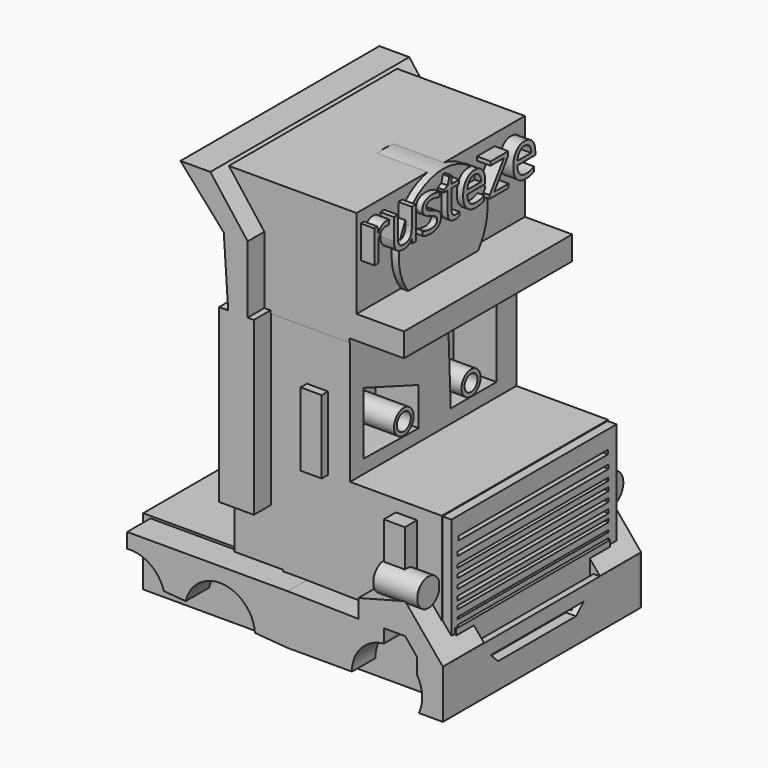
from build123d import *

# Parameters (mm, degrees)
F1_DEPTH       = 38.862
F1_DEPTH_BACK  = 39.878
F2_W           = 20.1118066907
F2_H           = 32.6452478766
F2_W_2         = 7.5783613138
F3_DEPTH       = 31.242
F3_DEPTH_BACK  = 34.798
F4_W           = 6.7039392889
F4_H           = 21.5691800695
F5_DEPTH       = 36.068
F5_DEPTH_BACK  = 37.084
F6_W           = 6.7039350979
F6_H           = 23.3180318028
F7_DEPTH       = 33.782
F7_DEPTH_BACK  = 36.83
F8_W           = 15.4481963255
F8_H           = 23.6095087603
F8_H_2         = 47.5104935467
F9_DEPTH       = 31.242
F9_DEPTH_BACK  = 35.052
F11_DEPTH      = 38.1
F11_DEPTH_BACK = 40.894
F13_DEPTH      = 31.496
F13_DEPTH_BACK = 35.306
F14_W          = 46.0130926222
F14_H          = 31.2351649627
F15_DEPTH      = 104.902
F15_DEPTH_BACK = 66.294
F16_R          = 11.155404916
F17_DEPTH      = 52.578
F17_DEPTH_BACK = 51.308
F18_R          = 3.81
F19_DEPTH      = 49.022
F19_DEPTH_BACK = 51.562
F20_DEPTH      = 25.4
F21_TEXT_SIZE  = 19.3375005654
F22_DEPTH      = 4.318
F23_R          = 17.6319533446
F24_DEPTH      = 18.288
F26_DEPTH      = 29.718
F27_R          = 3.8767676241
F27_R_2        = 2.7666686099
F27_R_3        = 3.7900369815
F27_R_4        = 2.5845106844
F28_DEPTH      = 13.716
F30_START      = 27.94
F29_R          = 4.4370042328
F29_R_2        = 4.9895919821
F30_DEPTH      = 13.97
F32_START      = 42.418
F31_W          = 65.579129383
F31_H          = 43.979652226
F32_DEPTH      = 3.302
F33_W          = 59.333499521
F33_H          = 1.3011721894
F33_W_2        = 60.1142030209
F33_H_2        = 1.3011731207
F33_H_3        = 0.9682839736
F33_H_4        = 1.1880891398
F33_H_5        = 1.1880899547
F33_H_6        = 1.2545959326
F33_H_7        = 1.0560783558
F33_H_8        = 0.660049729
F33_H_9        = 0.765087083
F34_DEPTH      = 11.176
F34_DEPTH_BACK = 4.064
F35_DEPTH      = 14.478
F37_START      = 47.244
F36_W          = 77.5241665542
F36_H          = 24.3252208456
F37_DEPTH      = 2.032
F38_W          = 9.0682730079
F38_H          = 14.4420657307
F39_DEPTH      = 40.894
F39_DEPTH_BACK = 39.37
F40_W          = 103.7813574076
F40_H          = 8.3965491503
F41_DEPTH      = 22.606
F41_DEPTH_BACK = 24.13
F42_W          = 36.1429508775
F42_H          = 4.5344494283
F43_DEPTH      = 0.254
F43_DEPTH_BACK = 66.04
F44_R          = 1.27
F45_DEPTH      = 41.91
F47_START      = 44.704
F47_DEPTH      = 21.336
F48_W          = 46.3489554822
F48_H          = 29.5391734689
F49_DEPTH      = 22.86
F51_START      = -8.636
F50_W          = 99.3931107223
F50_H          = 61.2098351121
F51_DEPTH      = 21.336


# Not quite as in the source:
# - Text() gives the source's letters only with a copy of the font that has no kerning and outlines rounded to 1/6400 em; it was checked with that copy


with BuildPart() as f1:
    # F0 (on Front) → F1 (new body, two sides)
    with BuildSketch(Plane.XZ) as f1_sk:
        Polygon((22.4436074495, -25.212623179), (30.3134415299, -25.212623179), (30.6049156934, -9.7644263878), (37.3088568449, -9.7644263878), (41.098035872, -14.4280325621), (41.098035872, -34.5398373902), (49.2593459785, -39.2034426332), (49.2593459785, -14.4280325621), (37.3088568449, 0), (22.4436074495, -3.9349179715), (22.4436074495, -9.7644263878), align=None)
        Polygon((0, -25.212623179), (22.4436074495, -25.212623179), (22.4436074495, -9.7644263878), (0, -9.3409639089), align=None)
        Polygon((-51.2313161539, -21.1662549384), (0, -25.212623179), (0, -9.3409639089), (-51.0081984103, -9.3409639089), align=None)
    extrude(amount=F1_DEPTH)
    extrude(f1_sk.sketch, amount=-F1_DEPTH_BACK)

    # F2 (on Front) → F3 (join, two sides)
    with BuildSketch(Plane.XZ) as f3_sk:
        with Locations((32.7909849584, 6.2667224556)):
            Rectangle(F2_W, F2_H)
        Polygon((0, -10.0559014827), (22.7350816131, -10.0559014827), (22.7350816131, 22.5893463939), (13.699343428, 22.5893463939), (0, 22.5893463939), align=None)
        with Locations((-3.7891806569, 6.2667224556)):
            Rectangle(F2_W_2, F2_H)
        Polygon((0, 22.5893463939), (13.699343428, 22.5893463939), (13.699343428, 61.6470463574), (-7.5783613138, 61.6470463574), (-7.5783613138, 22.5893463939), align=None)
    extrude(amount=F3_DEPTH)
    extrude(f3_sk.sketch, amount=-F3_DEPTH_BACK)

    # F4 (on Front) → F5 (join, two sides)
    with BuildSketch(Plane.XZ) as f5_sk:
        with Locations((31.6250827163, 8.0155736068)):
            Rectangle(F4_W, F4_H)
    extrude(amount=F5_DEPTH)
    extrude(f5_sk.sketch, amount=-F5_DEPTH_BACK)

    # F6 (on Front) → F7 (join, two sides)
    with BuildSketch(Plane.XZ) as f7_sk:
        with Locations((3.351967549, 33.9568844065)):
            Rectangle(F6_W, F6_H)
    extrude(amount=F7_DEPTH)
    extrude(f7_sk.sketch, amount=-F7_DEPTH_BACK)

    # F8 (on Front) → F9 (join, two sides)
    with BuildSketch(Plane.XZ) as f9_sk:
        with Locations((-15.3024594765, 2.9147542082)):
            Rectangle(F8_W, F8_H)
        with Locations((-15.3024594765, 38.4747553617)):
            Rectangle(F8_W, F8_H_2)
    extrude(amount=F9_DEPTH)
    extrude(f9_sk.sketch, amount=-F9_DEPTH_BACK)

    # F10 (on Front) → F11 (join, two sides)
    with BuildSketch(Plane.XZ) as f11_sk:
        Polygon((-22.4436074495, 8.0155739561), (-19.5288527757, 8.0155739561), (-11.3675408065, 8.0155739561), (-11.3675408065, 62.5214800239), (-13.3357383311, 62.5214800239), (-19.5288527757, 62.5214800239), (-22.4436074495, 62.5214800239), align=None)
        Polygon((-19.5288527757, 62.5214800239), (-13.3357383311, 62.5214800239), (-13.3357383311, 83.8632509112), (-25.2018421888, 99.4078442454), (-34.6947275102, 99.4078442454), (-20.930044353, 83.8632509112), align=None)
    extrude(amount=F11_DEPTH)
    extrude(f11_sk.sketch, amount=-F11_DEPTH_BACK)

    # F12 (on Front) → F13 (join, two sides)
    with BuildSketch(Plane.XZ) as f13_sk:
        Polygon((-26.0340645909, 98.6233502626), (-22.3627593368, 62.8767758608), (31.0406181961, 62.8767758608), (31.0406181961, 70.4034268856), (15.9873198718, 70.4034268856), (15.9873198718, 98.6233502626), align=None)
    extrude(amount=F13_DEPTH)
    extrude(f13_sk.sketch, amount=-F13_DEPTH_BACK)

    # F14 (on Right) → F15 (cut, two sides)
    with BuildSketch(Plane.YZ) as f15_sk:
        with Locations((0.5037942901, -23.661587853)):
            Rectangle(F14_W, F14_H)
    extrude(amount=-F15_DEPTH, mode=Mode.SUBTRACT)
    extrude(f15_sk.sketch, amount=F15_DEPTH_BACK, mode=Mode.SUBTRACT)

    # F16 (on Front) → F17 (cut, two sides)
    with BuildSketch(Plane.XZ) as f17_sk:
        with Locations((-50.0881457906, -25.1729656011)):
            Circle(F16_R)
        with Locations((-21.5410733944, -25.1729656011)):
            Circle(F16_R)
        with Locations((31.5516834733, -25.1729656011)):
            Circle(F16_R)
    extrude(amount=F17_DEPTH, mode=Mode.SUBTRACT)
    extrude(f17_sk.sketch, amount=-F17_DEPTH_BACK, mode=Mode.SUBTRACT)

    # F18 (on Front) → F19 (cut, two sides)
    with BuildSketch(Plane.XZ) as f19_sk:
        with Locations((31.6758154928, -25.5088303238)):
            Circle(F18_R)
        with Locations((-21.195452692, -25.5088303238)):
            Circle(F18_R)
        with Locations((-49.4832669438, -25.5088303238)):
            Circle(F18_R)
    extrude(amount=F19_DEPTH, mode=Mode.SUBTRACT)
    extrude(f19_sk.sketch, amount=-F19_DEPTH_BACK, mode=Mode.SUBTRACT)

    # F21 (on face) → F22 (join)
    with BuildSketch(Plane.YZ.offset(15.9873198718)):
        with Locations((-31.496, 84.7003498556)):
            Text('rusteze', F21_TEXT_SIZE, font='Open Sans', text_align=(TextAlign.LEFT, TextAlign.BOTTOM))
    extrude(amount=F22_DEPTH)

    # F23 (on Right) → F24 (join)
    with BuildSketch(Plane.YZ):
        with Locations((0, 81.2952890992)):
            Circle(F23_R)
    extrude(amount=F24_DEPTH)

    # F25 (on Right) → F26 (cut)
    with BuildSketch(Plane.YZ):
        Polygon((-25.8613731712, 46.7014983296), (-25.8613731712, 26.8856417388), (-4.0303440765, 26.5497807413), (-4.0303440765, 38.6408120394), align=None)
        Polygon((26.8689598888, 51.4035709202), (7.7248266898, 51.4035709202), (8.7324120104, 26.8856417388), (26.8689598888, 26.8856417388), align=None)
    extrude(amount=F26_DEPTH, mode=Mode.SUBTRACT)

    # F27 (on Right) → F28 (join)
    with BuildSketch(Plane.YZ):
        with Locations((-9.9086053669, 30.7821407914)):
            Circle(F27_R)
        with Locations((-9.9086053669, 30.7821407914)):
            Circle(F27_R_2, mode=Mode.SUBTRACT)
        with Locations((16.7778413743, 30.7821407914)):
            Circle(F27_R_3)
        with Locations((16.7778413743, 30.7821407914)):
            Circle(F27_R_4, mode=Mode.SUBTRACT)
    extrude(amount=F28_DEPTH)

    # F29 (on Right) → F30 (join)
    with BuildSketch(Plane.YZ.offset(F30_START)):
        with Locations((-35.3950075805, 2.5815158151)):
            Circle(F29_R)
        with Locations((37.0169132948, 1.7986835446)):
            Circle(F29_R_2)
    extrude(amount=F30_DEPTH)

    # F31 (on Right) → F32 (join)
    with BuildSketch(Plane.YZ.offset(F32_START)):
        with Locations((1.7691263929, 0.3647468984)):
            Rectangle(F31_W, F31_H)
    extrude(amount=F32_DEPTH)

    # F33 (on face) → F34 (cut, two sides)
    with BuildSketch(Plane.YZ.offset(45.72)) as f34_sk:
        with Locations((1.5088934451, 15.9788248129)):
            Rectangle(F33_W, F33_H)
        with Locations((1.3787755743, 11.815071106)):
            Rectangle(F33_W_2, F33_H_2)
        with Locations((1.3787755743, 8.3382311277)):
            Rectangle(F33_W_2, F33_H_3)
        with Locations((1.3787755743, 5.5439155549)):
            Rectangle(F33_W_2, F33_H_4)
        with Locations((1.3787755743, 2.5076873717)):
            Rectangle(F33_W_2, F33_H_5)
        with Locations((1.3787755743, -0.6272979663)):
            Rectangle(F33_W_2, F33_H_6)
        with Locations((1.3787755743, -3.234744072)):
            Rectangle(F33_W_2, F33_H_7)
        with Locations((1.3787755743, -6.2049669214)):
            Rectangle(F33_W_2, F33_H_8)
        with Locations((1.3787755743, -8.5016544908)):
            Rectangle(F33_W_2, F33_H_9)
    extrude(amount=F34_DEPTH, mode=Mode.SUBTRACT)
    extrude(f34_sk.sketch, amount=-F34_DEPTH_BACK, mode=Mode.SUBTRACT)

    # F33 (on face) → F35 (cut)
    with BuildSketch(Plane.YZ.offset(45.72)):
        with Locations((1.5088934451, 15.9788248129)):
            Rectangle(F33_W, F33_H)
        with Locations((1.3787755743, 11.815071106)):
            Rectangle(F33_W_2, F33_H_2)
        with Locations((1.3787755743, 8.3382311277)):
            Rectangle(F33_W_2, F33_H_3)
        with Locations((1.3787755743, 5.5439155549)):
            Rectangle(F33_W_2, F33_H_4)
        with Locations((1.3787755743, 2.5076873717)):
            Rectangle(F33_W_2, F33_H_5)
        with Locations((1.3787755743, -0.6272979663)):
            Rectangle(F33_W_2, F33_H_6)
        with Locations((1.3787755743, -3.234744072)):
            Rectangle(F33_W_2, F33_H_7)
        with Locations((1.3787755743, -6.2049669214)):
            Rectangle(F33_W_2, F33_H_8)
        with Locations((1.3787755743, -8.5016544908)):
            Rectangle(F33_W_2, F33_H_9)
    extrude(amount=F35_DEPTH, mode=Mode.SUBTRACT)

    # F36 (on Right) → F37 (join)
    with BuildSketch(Plane.YZ.offset(F37_START)):
        with Locations((0.2137403935, -26.6709891148)):
            Rectangle(F36_W, F36_H)
    extrude(amount=F37_DEPTH)

    # F38 (on Front) → F39 (cut, two sides)
    with BuildSketch(Plane.XZ) as f39_sk:
        with Locations((45.509301126, -37.0960673317)):
            Rectangle(F38_W, F38_H)
    extrude(amount=-F39_DEPTH, mode=Mode.SUBTRACT)
    extrude(f39_sk.sketch, amount=F39_DEPTH_BACK, mode=Mode.SUBTRACT)



with BuildPart() as f20:
    # F18 (on Front) → F20 (new body)
    with BuildSketch(Plane.XZ):
        with Locations((31.6758154928, -25.5088303238)):
            Circle(F18_R)
    extrude(amount=F20_DEPTH)


with BuildPart() as f20b:
    # F18 (on Front) → F20, piece 2 (new body)
    with BuildSketch(Plane.XZ):
        with Locations((-21.195452692, -25.5088303238)):
            Circle(F18_R)
    extrude(amount=F20_DEPTH)


with BuildPart() as f20c:
    # F18 (on Front) → F20, piece 3 (new body)
    with BuildSketch(Plane.XZ):
        with Locations((-49.4832669438, -25.5088303238)):
            Circle(F18_R)
    extrude(amount=F20_DEPTH)


with BuildPart() as f1_1:
    add(f1.part)

    add(f20.part)  # F41 merges F20

    add(f20b.part)  # F41 merges F20b

    add(f20c.part)  # F41 merges F20c
    # F40 (on Front) → F41 (join, two sides)
    with BuildSketch(Plane.XZ) as f41_sk:
        with Locations((-2.8548277915, -25.3408988938)):
            Rectangle(F40_W, F40_H)
    extrude(amount=F41_DEPTH)
    extrude(f41_sk.sketch, amount=-F41_DEPTH_BACK)

    # F42 (on face) → F43 (join, two sides)
    with BuildSketch(Plane.XZ.offset(31.242)) as f43_sk:
        with Locations((-4.3721320108, 63.9142710716)):
            Rectangle(F42_W, F42_H)
    extrude(amount=F43_DEPTH)
    extrude(f43_sk.sketch, amount=-F43_DEPTH_BACK)

    # F44 (on Top) → F45 (cut)
    with BuildSketch(Plane.XY):
        with Locations((-49.6846586466, -44.1644895208)):
            Circle(F44_R)
        with Locations((-21.6914974153, -44.1644895208)):
            Circle(F44_R)
        with Locations((32.0553742349, -44.1644895208)):
            Circle(F44_R)
        with Locations((-49.3211485445, 46.0860687625)):
            Circle(F44_R)
        with Locations((-20.8926349878, 46.0860687625)):
            Circle(F44_R)
        with Locations((32.0030450821, 46.0860687625)):
            Circle(F44_R)
    extrude(amount=-F45_DEPTH, mode=Mode.SUBTRACT)

    # F46 (on Right) → F47 (cut)
    with BuildSketch(Plane.YZ.offset(F47_START)):
        Polygon((17.0752834529, -18.9234726131), (-19.8043119162, -18.9234726131), (-16.9225558639, -21.804407239), (14.0087492764, -21.804407239), align=None)
    extrude(amount=F47_DEPTH, mode=Mode.SUBTRACT)

    # F48 (on Right) → F49 (join)
    with BuildSketch(Plane.YZ):
        with Locations((0.6717238575, -14.7695867345)):
            Rectangle(F48_W, F48_H)
    extrude(amount=-F49_DEPTH)

    # F50 (on Top) → F51 (join)
    with BuildSketch(Plane.XY.offset(F51_START)):
        with Locations((-3.643443808, 1.0201632977)):
            Rectangle(F50_W, F50_H)
    extrude(amount=-F51_DEPTH)


solid = f1_1.part
